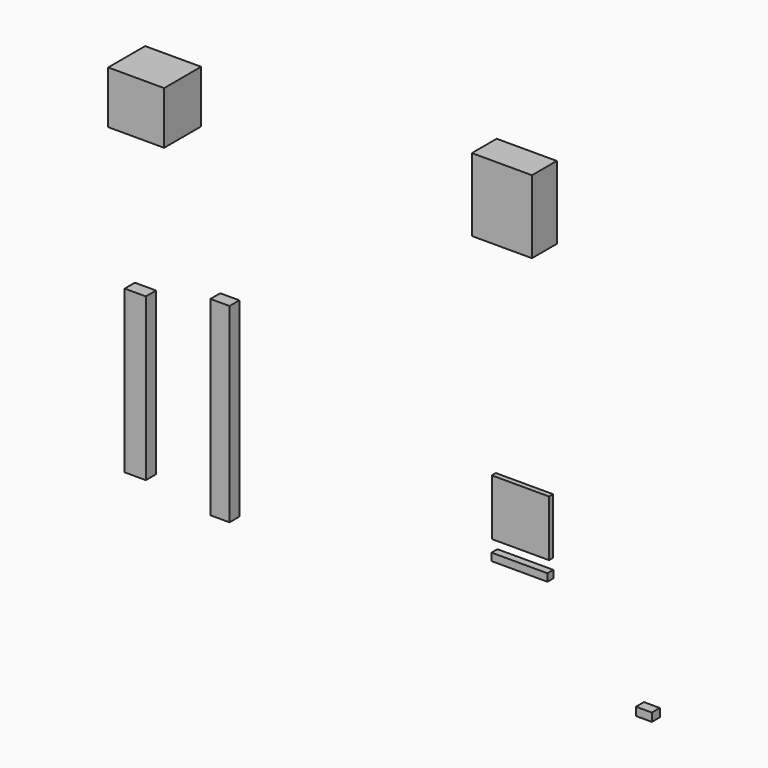
from build123d import *

# Parameters (mm, degrees)
F0_W      = 4.3286383152
F0_H      = 33.0931413919
F1_DEPTH  = 2.6221
F2_W      = 3.9097368717
F2_H      = 38.9577494934
F3_DEPTH  = 2.51867
F4_W      = 12.2877489775
F4_H      = 14.9407852441
F5_DEPTH  = 6.35
F6_W      = 11.4499479532
F6_H      = 10.7517801225
F7_DEPTH  = 9.45878
F8_W      = 11.7086973041
F8_H      = 11.4714205265
F9_DEPTH  = 1.02785
F12_W     = 11.4499498159
F12_H     = 1.5359669924
F13_DEPTH = 1.51179
F14_W     = 3.2493509352
F14_H     = 1.6868524253
F15_DEPTH = 2.03765


# Not quite as in the source:
# - the program builds the solid bodies; features that only make, move or delete a surface that nothing else refers to are left out


with BuildPart() as f1:
    # F0 (on Front) → F1 (new body)
    with BuildSketch(Plane.XZ):
        with Locations((-52.1531142294, -33.1629579887)):
            Rectangle(F0_W, F0_H)
    extrude(amount=F1_DEPTH)


with BuildPart() as f3:
    # F2 (on Front) → F3 (new body)
    with BuildSketch(Plane.XZ):
        with Locations((-34.9083766341, -32.32515743)):
            Rectangle(F2_W, F2_H)
    extrude(amount=F3_DEPTH)


with BuildPart() as f5:
    # F4 (on Front) → F5 (new body)
    with BuildSketch(Plane.XZ):
        with Locations((25.8321994916, 25.9020170197)):
            Rectangle(F4_W, F4_H)
    extrude(amount=F5_DEPTH)


with BuildPart() as f7:
    # F6 (on Front) → F7 (new body)
    with BuildSketch(Plane.XZ):
        with Locations((-46.4979596436, 21.2941113859)):
            Rectangle(F6_W, F6_H)
    extrude(amount=F7_DEPTH)


with BuildPart() as f9:
    # F8 (on Front) → F9 (new body)
    with BuildSketch(Plane.XZ):
        with Locations((25.358104147, -32.6233431697)):
            Rectangle(F8_W, F8_H)
    extrude(amount=F9_DEPTH)


with BuildPart() as f13:
    # F12 (on Front) → F13 (new body)
    with BuildSketch(Plane.XZ):
        with Locations((25.552934967, -41.261702776)):
            Rectangle(F12_W, F12_H)
    extrude(amount=F13_DEPTH)


with BuildPart() as f15:
    # F14 (on Front) → F15 (new body)
    with BuildSketch(Plane.XZ):
        with Locations((51.4326412231, -59.1236930341)):
            Rectangle(F14_W, F14_H)
    extrude(amount=F15_DEPTH)


solid = Compound([f1.part, f3.part, f5.part, f7.part, f9.part, f13.part, f15.part])
